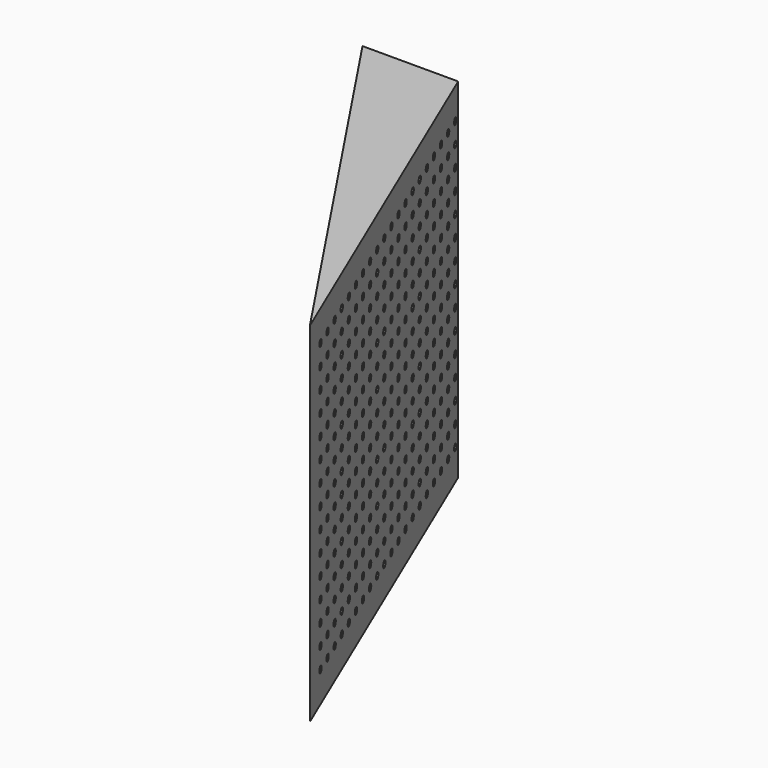
from build123d import *

# Parameters (mm, degrees)
F1_DEPTH      = 75
F2_DEPTH      = 5
F3_R          = 0.8
F4_DEPTH      = 17.9
F4_DEPTH_BACK = 4.1
F5_START      = 75
F5_DEPTH      = 5


# Not quite as in the source:
# - a feature names something its author has since deleted; it is built from what else it names


with BuildPart() as f1:
    # F0 (on Top) → F1 (new body)
    with BuildSketch(Plane.XY):
        Polygon((-89.710729354, 47.5730741788), (-88.2155505315, 45.3303059449), (-129.082574119, 141.6069801477), (-129.6257543077, 141.6069801477), align=None)
        Polygon((-91.2059081766, 49.8158424126), (-89.710729354, 47.5730741788), (-129.6257543077, 141.6069801477), (-130.1689344964, 141.6069801477), align=None)
    extrude(amount=F1_DEPTH)



with BuildPart() as f1b:
    # F0 (on Top) → F1, piece 2 (new body)
    with BuildSketch(Plane.XY):
        Polygon((-104.6625175797, 70.0007565173), (-103.1673387571, 67.7579882834), (-134.514376006, 141.6069801477), (-135.0575561947, 141.6069801477), align=None)
        Polygon((-106.1576964023, 72.2435247511), (-104.6625175797, 70.0007565173), (-135.0575561947, 141.6069801477), (-135.6007363834, 141.6069801477), align=None)
    extrude(amount=F1_DEPTH)


with BuildPart() as f1c:
    # F0 (on Top) → F1, piece 3 (new body)
    with BuildSketch(Plane.XY):
        Polygon((-119.6143058054, 92.4284388558), (-118.1191269828, 90.1856706219), (-139.946177893, 141.6069801477), (-140.4893580817, 141.6069801477), align=None)
        Polygon((-121.1094846279, 94.6712070896), (-119.6143058054, 92.4284388558), (-140.4893580817, 141.6069801477), (-141.0325382704, 141.6069801477), align=None)
    extrude(amount=F1_DEPTH)


with BuildPart() as f1d:
    # F0 (on Top) → F1, piece 4 (new body)
    with BuildSketch(Plane.XY):
        Polygon((-134.566094031, 114.8561211943), (-133.0709152085, 112.6133529604), (-145.3779797801, 141.6069801477), (-145.9211599688, 141.6069801477), align=None)
        Polygon((-136.0612728536, 117.0988894281), (-134.566094031, 114.8561211943), (-145.9211599688, 141.6069801477), (-146.4643401575, 141.6069801477), align=None)
    extrude(amount=F1_DEPTH)


with BuildPart() as f1_1:
    add(f1.part)

    add(f1b.part)  # F2 merges F1b

    add(f1c.part)  # F2 merges F1c

    add(f1d.part)  # F2 merges F1d
    # F0 (on Top) → F2 (join)
    with BuildSketch(Plane.XY):
        Polygon((-103.1673387571, 67.7579882834), (-91.2059081766, 49.8158424126), (-130.1689344964, 141.6069801477), (-134.514376006, 141.6069801477), align=None)
        Polygon((-89.710729354, 47.5730741788), (-88.2155505315, 45.3303059449), (-129.082574119, 141.6069801477), (-129.6257543077, 141.6069801477), align=None)
        Polygon((-91.2059081766, 49.8158424126), (-89.710729354, 47.5730741788), (-129.6257543077, 141.6069801477), (-130.1689344964, 141.6069801477), align=None)
        Polygon((-104.6625175797, 70.0007565173), (-103.1673387571, 67.7579882834), (-134.514376006, 141.6069801477), (-135.0575561947, 141.6069801477), align=None)
        Polygon((-106.1576964023, 72.2435247511), (-104.6625175797, 70.0007565173), (-135.0575561947, 141.6069801477), (-135.6007363834, 141.6069801477), align=None)
        Polygon((-118.1191269828, 90.1856706219), (-106.1576964023, 72.2435247511), (-135.6007363834, 141.6069801477), (-139.946177893, 141.6069801477), align=None)
        Polygon((-133.0709152085, 112.6133529604), (-121.1094846279, 94.6712070896), (-141.0325382704, 141.6069801477), (-145.3779797801, 141.6069801477), align=None)
        Polygon((-121.1094846279, 94.6712070896), (-119.6143058054, 92.4284388558), (-140.4893580817, 141.6069801477), (-141.0325382704, 141.6069801477), align=None)
        Polygon((-119.6143058054, 92.4284388558), (-118.1191269828, 90.1856706219), (-139.946177893, 141.6069801477), (-140.4893580817, 141.6069801477), align=None)
        Polygon((-134.566094031, 114.8561211943), (-133.0709152085, 112.6133529604), (-145.3779797801, 141.6069801477), (-145.9211599688, 141.6069801477), align=None)
        Polygon((-136.0612728536, 117.0988894281), (-134.566094031, 114.8561211943), (-145.9211599688, 141.6069801477), (-146.4643401575, 141.6069801477), align=None)
        Polygon((-152.4, 141.6069801477), (-136.0612728536, 117.0988894281), (-146.4643401575, 141.6069801477), align=None)
    extrude(amount=-F2_DEPTH)

    # F3 (on face) → F4 (cut, two sides)
    with BuildSketch(Plane(origin=(-59.364168796, -25.1985946391, 0), x_dir=(0.3907311285, -0.9205048535, 0), z_dir=(-0.9205048535, -0.3907311285, 0))) as f4_sk:
        with Locations((-178.7109671787, 2.5)):
            Circle(F3_R)
        with Locations((-178.7109671787, 7.5)):
            Circle(F3_R)
        with Locations((-178.7109671787, 12.5)):
            Circle(F3_R)
        with Locations((-178.7109671787, 17.5)):
            Circle(F3_R)
        with Locations((-178.7109671787, 22.5)):
            Circle(F3_R)
        with Locations((-178.7109671787, 27.5)):
            Circle(F3_R)
        with Locations((-178.7109671787, 32.5)):
            Circle(F3_R)
        with Locations((-178.7109671787, 37.5)):
            Circle(F3_R)
        with Locations((-178.7109671787, 42.5)):
            Circle(F3_R)
        with Locations((-178.7109671787, 47.5)):
            Circle(F3_R)
        with Locations((-178.7109671787, 52.5)):
            Circle(F3_R)
        with Locations((-178.7109671787, 57.5)):
            Circle(F3_R)
        with Locations((-178.7109671787, 62.5)):
            Circle(F3_R)
        with Locations((-178.7109671787, 67.5)):
            Circle(F3_R)
        with Locations((-178.7109671787, 72.5)):
            Circle(F3_R)
        with Locations((-173.7109671787, 2.5)):
            Circle(F3_R)
        with Locations((-173.7109671787, 7.5)):
            Circle(F3_R)
        with Locations((-173.7109671787, 12.5)):
            Circle(F3_R)
        with Locations((-173.7109671787, 17.5)):
            Circle(F3_R)
        with Locations((-173.7109671787, 22.5)):
            Circle(F3_R)
        with Locations((-173.7109671787, 27.5)):
            Circle(F3_R)
        with Locations((-173.7109671787, 32.5)):
            Circle(F3_R)
        with Locations((-173.7109671787, 37.5)):
            Circle(F3_R)
        with Locations((-173.7109671787, 42.5)):
            Circle(F3_R)
        with Locations((-173.7109671787, 47.5)):
            Circle(F3_R)
        with Locations((-173.7109671787, 52.5)):
            Circle(F3_R)
        with Locations((-173.7109671787, 57.5)):
            Circle(F3_R)
        with Locations((-173.7109671787, 62.5)):
            Circle(F3_R)
        with Locations((-173.7109671787, 67.5)):
            Circle(F3_R)
        with Locations((-173.7109671787, 72.5)):
            Circle(F3_R)
        with Locations((-168.7109671787, 2.5)):
            Circle(F3_R)
        with Locations((-168.7109671787, 7.5)):
            Circle(F3_R)
        with Locations((-168.7109671787, 12.5)):
            Circle(F3_R)
        with Locations((-168.7109671787, 17.5)):
            Circle(F3_R)
        with Locations((-168.7109671787, 22.5)):
            Circle(F3_R)
        with Locations((-168.7109671787, 27.5)):
            Circle(F3_R)
        with Locations((-168.7109671787, 32.5)):
            Circle(F3_R)
        with Locations((-168.7109671787, 37.5)):
            Circle(F3_R)
        with Locations((-168.7109671787, 42.5)):
            Circle(F3_R)
        with Locations((-168.7109671787, 47.5)):
            Circle(F3_R)
        with Locations((-168.7109671787, 52.5)):
            Circle(F3_R)
        with Locations((-168.7109671787, 57.5)):
            Circle(F3_R)
        with Locations((-168.7109671787, 62.5)):
            Circle(F3_R)
        with Locations((-168.7109671787, 67.5)):
            Circle(F3_R)
        with Locations((-168.7109671787, 72.5)):
            Circle(F3_R)
        with Locations((-163.7109671787, 2.5)):
            Circle(F3_R)
        with Locations((-163.7109671787, 7.5)):
            Circle(F3_R)
        with Locations((-163.7109671787, 12.5)):
            Circle(F3_R)
        with Locations((-163.7109671787, 17.5)):
            Circle(F3_R)
        with Locations((-163.7109671787, 22.5)):
            Circle(F3_R)
        with Locations((-163.7109671787, 27.5)):
            Circle(F3_R)
        with Locations((-163.7109671787, 32.5)):
            Circle(F3_R)
        with Locations((-163.7109671787, 37.5)):
            Circle(F3_R)
        with Locations((-163.7109671787, 42.5)):
            Circle(F3_R)
        with Locations((-163.7109671787, 47.5)):
            Circle(F3_R)
        with Locations((-163.7109671787, 52.5)):
            Circle(F3_R)
        with Locations((-163.7109671787, 57.5)):
            Circle(F3_R)
        with Locations((-163.7109671787, 62.5)):
            Circle(F3_R)
        with Locations((-163.7109671787, 67.5)):
            Circle(F3_R)
        with Locations((-163.7109671787, 72.5)):
            Circle(F3_R)
        with Locations((-158.7109671787, 2.5)):
            Circle(F3_R)
        with Locations((-158.7109671787, 7.5)):
            Circle(F3_R)
        with Locations((-158.7109671787, 12.5)):
            Circle(F3_R)
        with Locations((-158.7109671787, 17.5)):
            Circle(F3_R)
        with Locations((-158.7109671787, 22.5)):
            Circle(F3_R)
        with Locations((-158.7109671787, 27.5)):
            Circle(F3_R)
        with Locations((-158.7109671787, 32.5)):
            Circle(F3_R)
        with Locations((-158.7109671787, 37.5)):
            Circle(F3_R)
        with Locations((-158.7109671787, 42.5)):
            Circle(F3_R)
        with Locations((-158.7109671787, 47.5)):
            Circle(F3_R)
        with Locations((-158.7109671787, 52.5)):
            Circle(F3_R)
        with Locations((-158.7109671787, 57.5)):
            Circle(F3_R)
        with Locations((-158.7109671787, 62.5)):
            Circle(F3_R)
        with Locations((-158.7109671787, 67.5)):
            Circle(F3_R)
        with Locations((-158.7109671787, 72.5)):
            Circle(F3_R)
        with Locations((-153.7109671787, 2.5)):
            Circle(F3_R)
        with Locations((-153.7109671787, 7.5)):
            Circle(F3_R)
        with Locations((-153.7109671787, 12.5)):
            Circle(F3_R)
        with Locations((-153.7109671787, 17.5)):
            Circle(F3_R)
        with Locations((-153.7109671787, 22.5)):
            Circle(F3_R)
        with Locations((-153.7109671787, 27.5)):
            Circle(F3_R)
        with Locations((-153.7109671787, 32.5)):
            Circle(F3_R)
        with Locations((-153.7109671787, 37.5)):
            Circle(F3_R)
        with Locations((-153.7109671787, 42.5)):
            Circle(F3_R)
        with Locations((-153.7109671787, 47.5)):
            Circle(F3_R)
        with Locations((-153.7109671787, 52.5)):
            Circle(F3_R)
        with Locations((-153.7109671787, 57.5)):
            Circle(F3_R)
        with Locations((-153.7109671787, 62.5)):
            Circle(F3_R)
        with Locations((-153.7109671787, 67.5)):
            Circle(F3_R)
        with Locations((-153.7109671787, 72.5)):
            Circle(F3_R)
        with Locations((-148.7109671787, 2.5)):
            Circle(F3_R)
        with Locations((-148.7109671787, 7.5)):
            Circle(F3_R)
        with Locations((-148.7109671787, 12.5)):
            Circle(F3_R)
        with Locations((-148.7109671787, 17.5)):
            Circle(F3_R)
        with Locations((-148.7109671787, 22.5)):
            Circle(F3_R)
        with Locations((-148.7109671787, 27.5)):
            Circle(F3_R)
        with Locations((-148.7109671787, 32.5)):
            Circle(F3_R)
        with Locations((-148.7109671787, 37.5)):
            Circle(F3_R)
        with Locations((-148.7109671787, 42.5)):
            Circle(F3_R)
        with Locations((-148.7109671787, 47.5)):
            Circle(F3_R)
        with Locations((-148.7109671787, 52.5)):
            Circle(F3_R)
        with Locations((-148.7109671787, 57.5)):
            Circle(F3_R)
        with Locations((-148.7109671787, 62.5)):
            Circle(F3_R)
        with Locations((-148.7109671787, 67.5)):
            Circle(F3_R)
        with Locations((-148.7109671787, 72.5)):
            Circle(F3_R)
        with Locations((-143.7109671787, 2.5)):
            Circle(F3_R)
        with Locations((-143.7109671787, 7.5)):
            Circle(F3_R)
        with Locations((-143.7109671787, 12.5)):
            Circle(F3_R)
        with Locations((-143.7109671787, 17.5)):
            Circle(F3_R)
        with Locations((-143.7109671787, 22.5)):
            Circle(F3_R)
        with Locations((-143.7109671787, 27.5)):
            Circle(F3_R)
        with Locations((-143.7109671787, 32.5)):
            Circle(F3_R)
        with Locations((-143.7109671787, 37.5)):
            Circle(F3_R)
        with Locations((-143.7109671787, 42.5)):
            Circle(F3_R)
        with Locations((-143.7109671787, 47.5)):
            Circle(F3_R)
        with Locations((-143.7109671787, 52.5)):
            Circle(F3_R)
        with Locations((-143.7109671787, 57.5)):
            Circle(F3_R)
        with Locations((-143.7109671787, 62.5)):
            Circle(F3_R)
        with Locations((-143.7109671787, 67.5)):
            Circle(F3_R)
        with Locations((-143.7109671787, 72.5)):
            Circle(F3_R)
        with Locations((-138.7109671787, 2.5)):
            Circle(F3_R)
        with Locations((-138.7109671787, 7.5)):
            Circle(F3_R)
        with Locations((-138.7109671787, 12.5)):
            Circle(F3_R)
        with Locations((-138.7109671787, 17.5)):
            Circle(F3_R)
        with Locations((-138.7109671787, 22.5)):
            Circle(F3_R)
        with Locations((-138.7109671787, 27.5)):
            Circle(F3_R)
        with Locations((-138.7109671787, 32.5)):
            Circle(F3_R)
        with Locations((-138.7109671787, 37.5)):
            Circle(F3_R)
        with Locations((-138.7109671787, 42.5)):
            Circle(F3_R)
        with Locations((-138.7109671787, 47.5)):
            Circle(F3_R)
        with Locations((-138.7109671787, 52.5)):
            Circle(F3_R)
        with Locations((-138.7109671787, 57.5)):
            Circle(F3_R)
        with Locations((-138.7109671787, 62.5)):
            Circle(F3_R)
        with Locations((-138.7109671787, 67.5)):
            Circle(F3_R)
        with Locations((-138.7109671787, 72.5)):
            Circle(F3_R)
        with Locations((-133.7109671787, 2.5)):
            Circle(F3_R)
        with Locations((-133.7109671787, 7.5)):
            Circle(F3_R)
        with Locations((-133.7109671787, 12.5)):
            Circle(F3_R)
        with Locations((-133.7109671787, 17.5)):
            Circle(F3_R)
        with Locations((-133.7109671787, 22.5)):
            Circle(F3_R)
        with Locations((-133.7109671787, 27.5)):
            Circle(F3_R)
        with Locations((-133.7109671787, 32.5)):
            Circle(F3_R)
        with Locations((-133.7109671787, 37.5)):
            Circle(F3_R)
        with Locations((-133.7109671787, 42.5)):
            Circle(F3_R)
        with Locations((-133.7109671787, 47.5)):
            Circle(F3_R)
        with Locations((-133.7109671787, 52.5)):
            Circle(F3_R)
        with Locations((-133.7109671787, 57.5)):
            Circle(F3_R)
        with Locations((-133.7109671787, 62.5)):
            Circle(F3_R)
        with Locations((-133.7109671787, 67.5)):
            Circle(F3_R)
        with Locations((-133.7109671787, 72.5)):
            Circle(F3_R)
        with Locations((-128.7109671787, 2.5)):
            Circle(F3_R)
        with Locations((-128.7109671787, 7.5)):
            Circle(F3_R)
        with Locations((-128.7109671787, 12.5)):
            Circle(F3_R)
        with Locations((-128.7109671787, 17.5)):
            Circle(F3_R)
        with Locations((-128.7109671787, 22.5)):
            Circle(F3_R)
        with Locations((-128.7109671787, 27.5)):
            Circle(F3_R)
        with Locations((-128.7109671787, 32.5)):
            Circle(F3_R)
        with Locations((-128.7109671787, 37.5)):
            Circle(F3_R)
        with Locations((-128.7109671787, 42.5)):
            Circle(F3_R)
        with Locations((-128.7109671787, 47.5)):
            Circle(F3_R)
        with Locations((-128.7109671787, 52.5)):
            Circle(F3_R)
        with Locations((-128.7109671787, 57.5)):
            Circle(F3_R)
        with Locations((-128.7109671787, 62.5)):
            Circle(F3_R)
        with Locations((-128.7109671787, 67.5)):
            Circle(F3_R)
        with Locations((-128.7109671787, 72.5)):
            Circle(F3_R)
        with Locations((-123.7109671787, 2.5)):
            Circle(F3_R)
        with Locations((-123.7109671787, 7.5)):
            Circle(F3_R)
        with Locations((-123.7109671787, 12.5)):
            Circle(F3_R)
        with Locations((-123.7109671787, 17.5)):
            Circle(F3_R)
        with Locations((-123.7109671787, 22.5)):
            Circle(F3_R)
        with Locations((-123.7109671787, 27.5)):
            Circle(F3_R)
        with Locations((-123.7109671787, 32.5)):
            Circle(F3_R)
        with Locations((-123.7109671787, 37.5)):
            Circle(F3_R)
        with Locations((-123.7109671787, 42.5)):
            Circle(F3_R)
        with Locations((-123.7109671787, 47.5)):
            Circle(F3_R)
        with Locations((-123.7109671787, 52.5)):
            Circle(F3_R)
        with Locations((-123.7109671787, 57.5)):
            Circle(F3_R)
        with Locations((-123.7109671787, 62.5)):
            Circle(F3_R)
        with Locations((-123.7109671787, 67.5)):
            Circle(F3_R)
        with Locations((-123.7109671787, 72.5)):
            Circle(F3_R)
        with Locations((-118.7109671787, 2.5)):
            Circle(F3_R)
        with Locations((-118.7109671787, 7.5)):
            Circle(F3_R)
        with Locations((-118.7109671787, 12.5)):
            Circle(F3_R)
        with Locations((-118.7109671787, 17.5)):
            Circle(F3_R)
        with Locations((-118.7109671787, 22.5)):
            Circle(F3_R)
        with Locations((-118.7109671787, 27.5)):
            Circle(F3_R)
        with Locations((-118.7109671787, 32.5)):
            Circle(F3_R)
        with Locations((-118.7109671787, 37.5)):
            Circle(F3_R)
        with Locations((-118.7109671787, 42.5)):
            Circle(F3_R)
        with Locations((-118.7109671787, 47.5)):
            Circle(F3_R)
        with Locations((-118.7109671787, 52.5)):
            Circle(F3_R)
        with Locations((-118.7109671787, 57.5)):
            Circle(F3_R)
        with Locations((-118.7109671787, 62.5)):
            Circle(F3_R)
        with Locations((-118.7109671787, 67.5)):
            Circle(F3_R)
        with Locations((-118.7109671787, 72.5)):
            Circle(F3_R)
        with Locations((-113.7109671787, 2.5)):
            Circle(F3_R)
        with Locations((-113.7109671787, 7.5)):
            Circle(F3_R)
        with Locations((-113.7109671787, 12.5)):
            Circle(F3_R)
        with Locations((-113.7109671787, 17.5)):
            Circle(F3_R)
        with Locations((-113.7109671787, 22.5)):
            Circle(F3_R)
        with Locations((-113.7109671787, 27.5)):
            Circle(F3_R)
        with Locations((-113.7109671787, 32.5)):
            Circle(F3_R)
        with Locations((-113.7109671787, 37.5)):
            Circle(F3_R)
        with Locations((-113.7109671787, 42.5)):
            Circle(F3_R)
        with Locations((-113.7109671787, 47.5)):
            Circle(F3_R)
        with Locations((-113.7109671787, 52.5)):
            Circle(F3_R)
        with Locations((-113.7109671787, 57.5)):
            Circle(F3_R)
        with Locations((-113.7109671787, 62.5)):
            Circle(F3_R)
        with Locations((-113.7109671787, 67.5)):
            Circle(F3_R)
        with Locations((-113.7109671787, 72.5)):
            Circle(F3_R)
        with Locations((-108.7109671787, 2.5)):
            Circle(F3_R)
        with Locations((-108.7109671787, 7.5)):
            Circle(F3_R)
        with Locations((-108.7109671787, 12.5)):
            Circle(F3_R)
        with Locations((-108.7109671787, 17.5)):
            Circle(F3_R)
        with Locations((-108.7109671787, 22.5)):
            Circle(F3_R)
        with Locations((-108.7109671787, 27.5)):
            Circle(F3_R)
        with Locations((-108.7109671787, 32.5)):
            Circle(F3_R)
        with Locations((-108.7109671787, 37.5)):
            Circle(F3_R)
        with Locations((-108.7109671787, 42.5)):
            Circle(F3_R)
        with Locations((-108.7109671787, 47.5)):
            Circle(F3_R)
        with Locations((-108.7109671787, 52.5)):
            Circle(F3_R)
        with Locations((-108.7109671787, 57.5)):
            Circle(F3_R)
        with Locations((-108.7109671787, 62.5)):
            Circle(F3_R)
        with Locations((-108.7109671787, 67.5)):
            Circle(F3_R)
        with Locations((-108.7109671787, 72.5)):
            Circle(F3_R)
        with Locations((-103.7109671787, 2.5)):
            Circle(F3_R)
        with Locations((-103.7109671787, 7.5)):
            Circle(F3_R)
        with Locations((-103.7109671787, 12.5)):
            Circle(F3_R)
        with Locations((-103.7109671787, 17.5)):
            Circle(F3_R)
        with Locations((-103.7109671787, 22.5)):
            Circle(F3_R)
        with Locations((-103.7109671787, 27.5)):
            Circle(F3_R)
        with Locations((-103.7109671787, 32.5)):
            Circle(F3_R)
        with Locations((-103.7109671787, 37.5)):
            Circle(F3_R)
        with Locations((-103.7109671787, 42.5)):
            Circle(F3_R)
        with Locations((-103.7109671787, 47.5)):
            Circle(F3_R)
        with Locations((-103.7109671787, 52.5)):
            Circle(F3_R)
        with Locations((-103.7109671787, 57.5)):
            Circle(F3_R)
        with Locations((-103.7109671787, 62.5)):
            Circle(F3_R)
        with Locations((-103.7109671787, 67.5)):
            Circle(F3_R)
        with Locations((-103.7109671787, 72.5)):
            Circle(F3_R)
        with Locations((-98.7109671787, 2.5)):
            Circle(F3_R)
        with Locations((-98.7109671787, 7.5)):
            Circle(F3_R)
        with Locations((-98.7109671787, 12.5)):
            Circle(F3_R)
        with Locations((-98.7109671787, 17.5)):
            Circle(F3_R)
        with Locations((-98.7109671787, 22.5)):
            Circle(F3_R)
        with Locations((-98.7109671787, 27.5)):
            Circle(F3_R)
        with Locations((-98.7109671787, 32.5)):
            Circle(F3_R)
        with Locations((-98.7109671787, 37.5)):
            Circle(F3_R)
        with Locations((-98.7109671787, 42.5)):
            Circle(F3_R)
        with Locations((-98.7109671787, 47.5)):
            Circle(F3_R)
        with Locations((-98.7109671787, 52.5)):
            Circle(F3_R)
        with Locations((-98.7109671787, 57.5)):
            Circle(F3_R)
        with Locations((-98.7109671787, 62.5)):
            Circle(F3_R)
        with Locations((-98.7109671787, 67.5)):
            Circle(F3_R)
        with Locations((-98.7109671787, 72.5)):
            Circle(F3_R)
        with Locations((-93.7109671787, 2.5)):
            Circle(F3_R)
        with Locations((-93.7109671787, 7.5)):
            Circle(F3_R)
        with Locations((-93.7109671787, 12.5)):
            Circle(F3_R)
        with Locations((-93.7109671787, 17.5)):
            Circle(F3_R)
        with Locations((-93.7109671787, 22.5)):
            Circle(F3_R)
        with Locations((-93.7109671787, 27.5)):
            Circle(F3_R)
        with Locations((-93.7109671787, 32.5)):
            Circle(F3_R)
        with Locations((-93.7109671787, 37.5)):
            Circle(F3_R)
        with Locations((-93.7109671787, 42.5)):
            Circle(F3_R)
        with Locations((-93.7109671787, 47.5)):
            Circle(F3_R)
        with Locations((-93.7109671787, 52.5)):
            Circle(F3_R)
        with Locations((-93.7109671787, 57.5)):
            Circle(F3_R)
        with Locations((-93.7109671787, 62.5)):
            Circle(F3_R)
        with Locations((-93.7109671787, 67.5)):
            Circle(F3_R)
        with Locations((-93.7109671787, 72.5)):
            Circle(F3_R)
        with Locations((-88.7109671787, 2.5)):
            Circle(F3_R)
        with Locations((-88.7109671787, 7.5)):
            Circle(F3_R)
        with Locations((-88.7109671787, 12.5)):
            Circle(F3_R)
        with Locations((-88.7109671787, 17.5)):
            Circle(F3_R)
        with Locations((-88.7109671787, 22.5)):
            Circle(F3_R)
        with Locations((-88.7109671787, 27.5)):
            Circle(F3_R)
        with Locations((-88.7109671787, 32.5)):
            Circle(F3_R)
        with Locations((-88.7109671787, 37.5)):
            Circle(F3_R)
        with Locations((-88.7109671787, 42.5)):
            Circle(F3_R)
        with Locations((-88.7109671787, 47.5)):
            Circle(F3_R)
        with Locations((-88.7109671787, 52.5)):
            Circle(F3_R)
        with Locations((-88.7109671787, 57.5)):
            Circle(F3_R)
        with Locations((-88.7109671787, 62.5)):
            Circle(F3_R)
        with Locations((-88.7109671787, 67.5)):
            Circle(F3_R)
        with Locations((-88.7109671787, 72.5)):
            Circle(F3_R)
        with Locations((-83.7109671787, 2.5)):
            Circle(F3_R)
        with Locations((-83.7109671787, 7.5)):
            Circle(F3_R)
        with Locations((-83.7109671787, 12.5)):
            Circle(F3_R)
        with Locations((-83.7109671787, 17.5)):
            Circle(F3_R)
        with Locations((-83.7109671787, 22.5)):
            Circle(F3_R)
        with Locations((-83.7109671787, 27.5)):
            Circle(F3_R)
        with Locations((-83.7109671787, 32.5)):
            Circle(F3_R)
        with Locations((-83.7109671787, 37.5)):
            Circle(F3_R)
        with Locations((-83.7109671787, 42.5)):
            Circle(F3_R)
        with Locations((-83.7109671787, 47.5)):
            Circle(F3_R)
        with Locations((-83.7109671787, 52.5)):
            Circle(F3_R)
        with Locations((-83.7109671787, 57.5)):
            Circle(F3_R)
        with Locations((-83.7109671787, 62.5)):
            Circle(F3_R)
        with Locations((-83.7109671787, 67.5)):
            Circle(F3_R)
        with Locations((-83.7109671787, 72.5)):
            Circle(F3_R)
        with Locations((-183.7109671787, 72.5)):
            Circle(F3_R)
        with Locations((-183.7109671787, 67.5)):
            Circle(F3_R)
        with Locations((-183.7109671787, 62.5)):
            Circle(F3_R)
        with Locations((-183.7109671787, 57.5)):
            Circle(F3_R)
        with Locations((-183.7109671787, 52.5)):
            Circle(F3_R)
        with Locations((-183.7109671787, 47.5)):
            Circle(F3_R)
        with Locations((-183.7109671787, 42.5)):
            Circle(F3_R)
        with Locations((-183.7109671787, 37.5)):
            Circle(F3_R)
        with Locations((-183.7109671787, 32.5)):
            Circle(F3_R)
        with Locations((-183.7109671787, 27.5)):
            Circle(F3_R)
        with Locations((-183.7109671787, 22.5)):
            Circle(F3_R)
        with Locations((-183.7109671787, 17.5)):
            Circle(F3_R)
        with Locations((-183.7109671787, 12.5)):
            Circle(F3_R)
        with Locations((-183.7109671787, 7.5)):
            Circle(F3_R)
        with Locations((-183.7109671787, 2.5)):
            Circle(F3_R)
        with Locations((-188.7109671787, 72.5)):
            Circle(F3_R)
        with Locations((-188.7109671787, 67.5)):
            Circle(F3_R)
        with Locations((-188.7109671787, 62.5)):
            Circle(F3_R)
        with Locations((-188.7109671787, 57.5)):
            Circle(F3_R)
        with Locations((-188.7109671787, 52.5)):
            Circle(F3_R)
        with Locations((-188.7109671787, 47.5)):
            Circle(F3_R)
        with Locations((-188.7109671787, 42.5)):
            Circle(F3_R)
        with Locations((-188.7109671787, 37.5)):
            Circle(F3_R)
        with Locations((-188.7109671787, 32.5)):
            Circle(F3_R)
        with Locations((-188.7109671787, 27.5)):
            Circle(F3_R)
        with Locations((-188.7109671787, 22.5)):
            Circle(F3_R)
        with Locations((-188.7109671787, 17.5)):
            Circle(F3_R)
        with Locations((-188.7109671787, 12.5)):
            Circle(F3_R)
        with Locations((-188.7109671787, 7.5)):
            Circle(F3_R)
        with Locations((-188.7109671787, 2.5)):
            Circle(F3_R)
        with Locations((-193.7109671787, 72.5)):
            Circle(F3_R)
        with Locations((-193.7109671787, 67.5)):
            Circle(F3_R)
        with Locations((-193.7109671787, 62.5)):
            Circle(F3_R)
        with Locations((-193.7109671787, 57.5)):
            Circle(F3_R)
        with Locations((-193.7109671787, 52.5)):
            Circle(F3_R)
        with Locations((-193.7109671787, 47.5)):
            Circle(F3_R)
        with Locations((-193.7109671787, 42.5)):
            Circle(F3_R)
        with Locations((-193.7109671787, 37.5)):
            Circle(F3_R)
        with Locations((-193.7109671787, 32.5)):
            Circle(F3_R)
        with Locations((-193.7109671787, 27.5)):
            Circle(F3_R)
        with Locations((-193.7109671787, 22.5)):
            Circle(F3_R)
        with Locations((-193.7109671787, 17.5)):
            Circle(F3_R)
        with Locations((-193.7109671787, 12.5)):
            Circle(F3_R)
        with Locations((-193.7109671787, 7.5)):
            Circle(F3_R)
        with Locations((-193.7109671787, 2.5)):
            Circle(F3_R)
        with Locations((-198.7109671787, 72.5)):
            Circle(F3_R)
        with Locations((-198.7109671787, 67.5)):
            Circle(F3_R)
        with Locations((-198.7109671787, 62.5)):
            Circle(F3_R)
        with Locations((-198.7109671787, 57.5)):
            Circle(F3_R)
        with Locations((-198.7109671787, 52.5)):
            Circle(F3_R)
        with Locations((-198.7109671787, 47.5)):
            Circle(F3_R)
        with Locations((-198.7109671787, 42.5)):
            Circle(F3_R)
        with Locations((-198.7109671787, 37.5)):
            Circle(F3_R)
        with Locations((-198.7109671787, 32.5)):
            Circle(F3_R)
        with Locations((-198.7109671787, 27.5)):
            Circle(F3_R)
        with Locations((-198.7109671787, 22.5)):
            Circle(F3_R)
        with Locations((-198.7109671787, 17.5)):
            Circle(F3_R)
        with Locations((-198.7109671787, 12.5)):
            Circle(F3_R)
        with Locations((-198.7109671787, 7.5)):
            Circle(F3_R)
        with Locations((-198.7109671787, 2.5)):
            Circle(F3_R)
    extrude(amount=F4_DEPTH, mode=Mode.SUBTRACT)
    extrude(f4_sk.sketch, amount=-F4_DEPTH_BACK, mode=Mode.SUBTRACT)

    # F0 (on Top) → F5 (join)
    with BuildSketch(Plane.XY.offset(F5_START)):
        Polygon((-103.1673387571, 67.7579882834), (-91.2059081766, 49.8158424126), (-130.1689344964, 141.6069801477), (-134.514376006, 141.6069801477), align=None)
        Polygon((-91.2059081766, 49.8158424126), (-89.710729354, 47.5730741788), (-129.6257543077, 141.6069801477), (-130.1689344964, 141.6069801477), align=None)
        Polygon((-89.710729354, 47.5730741788), (-88.2155505315, 45.3303059449), (-129.082574119, 141.6069801477), (-129.6257543077, 141.6069801477), align=None)
        Polygon((-106.1576964023, 72.2435247511), (-104.6625175797, 70.0007565173), (-135.0575561947, 141.6069801477), (-135.6007363834, 141.6069801477), align=None)
        Polygon((-104.6625175797, 70.0007565173), (-103.1673387571, 67.7579882834), (-134.514376006, 141.6069801477), (-135.0575561947, 141.6069801477), align=None)
        Polygon((-152.4, 141.6069801477), (-136.0612728536, 117.0988894281), (-146.4643401575, 141.6069801477), align=None)
        Polygon((-118.1191269828, 90.1856706219), (-106.1576964023, 72.2435247511), (-135.6007363834, 141.6069801477), (-139.946177893, 141.6069801477), align=None)
        Polygon((-133.0709152085, 112.6133529604), (-121.1094846279, 94.6712070896), (-141.0325382704, 141.6069801477), (-145.3779797801, 141.6069801477), align=None)
        Polygon((-121.1094846279, 94.6712070896), (-119.6143058054, 92.4284388558), (-140.4893580817, 141.6069801477), (-141.0325382704, 141.6069801477), align=None)
        Polygon((-119.6143058054, 92.4284388558), (-118.1191269828, 90.1856706219), (-139.946177893, 141.6069801477), (-140.4893580817, 141.6069801477), align=None)
        Polygon((-134.566094031, 114.8561211943), (-133.0709152085, 112.6133529604), (-145.3779797801, 141.6069801477), (-145.9211599688, 141.6069801477), align=None)
        Polygon((-136.0612728536, 117.0988894281), (-134.566094031, 114.8561211943), (-145.9211599688, 141.6069801477), (-146.4643401575, 141.6069801477), align=None)
    extrude(amount=F5_DEPTH)


solid = f1_1.part
